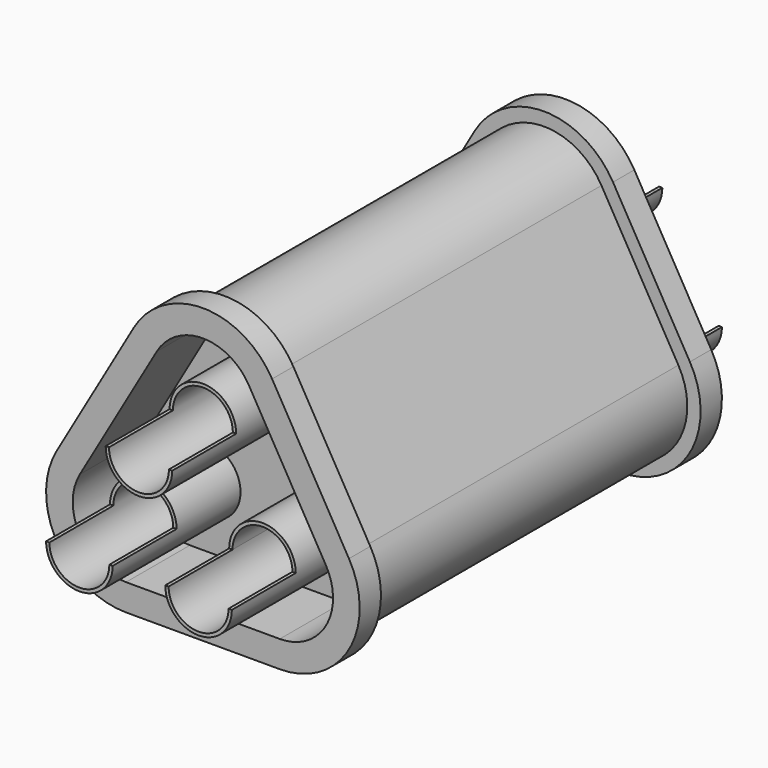
from build123d import *
from build123d import SkipClean  # not in build123d's __all__

# Parameters (mm, degrees)
F1_DEPTH  = 17
F2_DEPTH  = 1
F3_DEPTH  = 3
F4_DEPTH  = 17
F5_DEPTH  = 20
F6_DEPTH  = 14
F7_DEPTH  = 3
F8_DEPTH  = 3
F10_DEPTH = 1
F9_R      = 1.25
F11_DEPTH = 3


with BuildPart() as f1:
    # F0 (on Front) → F1 (new body)
    with BuildSketch(Plane.XZ):
        with BuildLine():
            Line((-2.1650635095, 3.4944827652), (-5.0518148554, -1.5055172348))
            ThreePointArc((-5.0518148554, -1.5055172348), (-5.0518148554, -4.0055172348), (-2.8867513459, -5.2555172348))
            Line((-2.8867513459, -5.2555172348), (2.8867513459, -5.2555172348))
            ThreePointArc((2.8867513459, -5.2555172348), (5.0518148554, -4.0055172348), (5.0518148554, -1.5055172348))
            Line((5.0518148554, -1.5055172348), (2.1650635095, 3.4944827652))
            ThreePointArc((2.1650635095, 3.4944827652), (0, 4.7444827652), (-2.1650635095, 3.4944827652))
        make_face()
        with BuildLine():
            ThreePointArc((-2.8867513459, -4.7555172348), (-4.6188021535, -3.7555172348), (-4.6188021535, -1.7555172348))
            Line((-4.6188021535, -1.7555172348), (-1.7320508076, 3.2444827652))
            ThreePointArc((-1.7320508076, 3.2444827652), (0, 4.2444827652), (1.7320508076, 3.2444827652))
            Line((1.7320508076, 3.2444827652), (4.6188021535, -1.7555172348))
            ThreePointArc((4.6188021535, -1.7555172348), (4.6188021535, -3.7555172348), (2.8867513459, -4.7555172348))
            Line((2.8867513459, -4.7555172348), (-2.8867513459, -4.7555172348))
        make_face(mode=Mode.SUBTRACT)
        with BuildLine():
            Line((-1.7320508076, 3.2444827652), (-4.6188021535, -1.7555172348))
            ThreePointArc((-4.6188021535, -1.7555172348), (-4.6188021535, -3.7555172348), (-2.8867513459, -4.7555172348))
            Line((-2.8867513459, -4.7555172348), (2.8867513459, -4.7555172348))
            ThreePointArc((2.8867513459, -4.7555172348), (4.6188021535, -3.7555172348), (4.6188021535, -1.7555172348))
            Line((4.6188021535, -1.7555172348), (1.7320508076, 3.2444827652))
            ThreePointArc((1.7320508076, 3.2444827652), (0, 4.2444827652), (-1.7320508076, 3.2444827652))
        make_face()
        with BuildLine():
            ThreePointArc((-3.4872322931, -2.3805172348), (-2.2372322931, -1.1305172348), (-0.9872322931, -2.3805172348))
            ThreePointArc((-0.9872322931, -2.3805172348), (-2.2372322931, -3.6305172348), (-3.4872322931, -2.3805172348))
        make_face(mode=Mode.SUBTRACT)
        with BuildLine():
            ThreePointArc((0.9872322931, -2.3805172348), (2.2372322931, -1.1305172348), (3.4872322931, -2.3805172348))
            ThreePointArc((3.4872322931, -2.3805172348), (2.2372322931, -3.6305172348), (0.9872322931, -2.3805172348))
        make_face(mode=Mode.SUBTRACT)
        with BuildLine():
            ThreePointArc((-1.25, 1.4944827652), (0, 2.7444827652), (1.25, 1.4944827652))
            ThreePointArc((1.25, 1.4944827652), (0, 0.2444827652), (-1.25, 1.4944827652))
        make_face(mode=Mode.SUBTRACT)
    extrude(amount=F1_DEPTH)

    # F0 (on Front) → F2 (join)
    with BuildSketch(Plane.XZ):
        with BuildLine():
            Line((-2.5980762114, 3.7444827652), (-5.4848275573, -1.2555172348))
            ThreePointArc((-5.4848275573, -1.2555172348), (-5.4848275573, -4.2555172348), (-2.8867513459, -5.7555172348))
            Line((-2.8867513459, -5.7555172348), (2.8867513459, -5.7555172348))
            ThreePointArc((2.8867513459, -5.7555172348), (5.4848275573, -4.2555172348), (5.4848275573, -1.2555172348))
            Line((5.4848275573, -1.2555172348), (2.5980762114, 3.7444827652))
            ThreePointArc((2.5980762114, 3.7444827652), (0, 5.2444827652), (-2.5980762114, 3.7444827652))
        make_face()
        with BuildLine():
            ThreePointArc((-2.8867513459, -5.2555172348), (-5.0518148554, -4.0055172348), (-5.0518148554, -1.5055172348))
            Line((-5.0518148554, -1.5055172348), (-2.1650635095, 3.4944827652))
            ThreePointArc((-2.1650635095, 3.4944827652), (0, 4.7444827652), (2.1650635095, 3.4944827652))
            Line((2.1650635095, 3.4944827652), (5.0518148554, -1.5055172348))
            ThreePointArc((5.0518148554, -1.5055172348), (5.0518148554, -4.0055172348), (2.8867513459, -5.2555172348))
            Line((2.8867513459, -5.2555172348), (-2.8867513459, -5.2555172348))
        make_face(mode=Mode.SUBTRACT)
    extrude(amount=F2_DEPTH)

    # F0 (on Front) → F3 (cut)
    with BuildSketch(Plane.XZ):
        with BuildLine():
            Line((-1.7320508076, 3.2444827652), (-4.6188021535, -1.7555172348))
            ThreePointArc((-4.6188021535, -1.7555172348), (-4.6188021535, -3.7555172348), (-2.8867513459, -4.7555172348))
            Line((-2.8867513459, -4.7555172348), (2.8867513459, -4.7555172348))
            ThreePointArc((2.8867513459, -4.7555172348), (4.6188021535, -3.7555172348), (4.6188021535, -1.7555172348))
            Line((4.6188021535, -1.7555172348), (1.7320508076, 3.2444827652))
            ThreePointArc((1.7320508076, 3.2444827652), (0, 4.2444827652), (-1.7320508076, 3.2444827652))
        make_face()
        with BuildLine():
            ThreePointArc((-3.4872322931, -2.3805172348), (-2.2372322931, -1.1305172348), (-0.9872322931, -2.3805172348))
            ThreePointArc((-0.9872322931, -2.3805172348), (-2.2372322931, -3.6305172348), (-3.4872322931, -2.3805172348))
        make_face(mode=Mode.SUBTRACT)
        with BuildLine():
            ThreePointArc((0.9872322931, -2.3805172348), (2.2372322931, -1.1305172348), (3.4872322931, -2.3805172348))
            ThreePointArc((3.4872322931, -2.3805172348), (2.2372322931, -3.6305172348), (0.9872322931, -2.3805172348))
        make_face(mode=Mode.SUBTRACT)
        with BuildLine():
            ThreePointArc((-1.25, 1.4944827652), (0, 2.7444827652), (1.25, 1.4944827652))
            ThreePointArc((1.25, 1.4944827652), (0, 0.2444827652), (-1.25, 1.4944827652))
        make_face(mode=Mode.SUBTRACT)
        with BuildLine():
            ThreePointArc((1.112232334, -2.3805172348), (2.2372322931, -3.5055171939), (3.3622322522, -2.3805172348))
            ThreePointArc((3.3622322522, -2.3805172348), (2.2372322931, -1.2555172756), (1.112232334, -2.3805172348))
        make_face()
        with BuildLine():
            ThreePointArc((-1.125, 1.4944827652), (0, 0.3694827652), (1.125, 1.4944827652))
            ThreePointArc((1.125, 1.4944827652), (0, 2.6194827652), (-1.125, 1.4944827652))
        make_face()
        with BuildLine():
            ThreePointArc((-3.3622322931, -2.3805172348), (-2.2372322931, -3.5055172348), (-1.1122322931, -2.3805172348))
            ThreePointArc((-1.1122322931, -2.3805172348), (-2.2372322931, -1.2555172348), (-3.3622322931, -2.3805172348))
        make_face()
    extrude(amount=F3_DEPTH, mode=Mode.SUBTRACT)

    # F9 (on face) → F10 (join)
    with BuildSketch(Plane.XZ.offset(17)):
        with BuildLine():
            Line((-2.5980762912, 3.7444828113), (-5.4848276371, -1.2555171887))
            ThreePointArc((-5.4848276371, -1.2555171887), (-5.4848276371, -4.2555172809), (-2.8867513459, -5.7555173269))
            Line((-2.8867513459, -5.7555173269), (2.8867513459, -5.7555173269))
            ThreePointArc((2.8867513459, -5.7555173269), (5.4848276371, -4.2555172809), (5.4848276371, -1.2555171887))
            Line((5.4848276371, -1.2555171887), (2.5980762912, 3.7444828113))
            ThreePointArc((2.5980762912, 3.7444828113), (0, 5.2444828574), (-2.5980762912, 3.7444828113))
        make_face()
        with BuildLine():
            Line((-5.0518148554, -1.5055172348), (-2.1650635095, 3.4944827652))
            ThreePointArc((-2.1650635095, 3.4944827652), (0, 4.7444827652), (2.1650635095, 3.4944827652))
            Line((2.1650635095, 3.4944827652), (5.0518148554, -1.5055172348))
            ThreePointArc((5.0518148554, -1.5055172348), (5.0518148554, -4.0055172348), (2.8867513459, -5.2555172348))
            Line((2.8867513459, -5.2555172348), (-2.8867513459, -5.2555172348))
            ThreePointArc((-2.8867513459, -5.2555172348), (-5.0518148554, -4.0055172348), (-5.0518148554, -1.5055172348))
        make_face(mode=Mode.SUBTRACT)
    extrude(amount=-F10_DEPTH)

    # F9 (on face) → F11 (cut)
    with BuildSketch(Plane.XZ.offset(17)):
        with BuildLine():
            Line((-1.7320508399, 3.2444827839), (-4.6188021858, -1.7555172161))
            ThreePointArc((-4.6188021858, -1.7555172161), (-4.6188021858, -3.7555172534), (-2.8867513459, -4.7555172721))
            Line((-2.8867513459, -4.7555172721), (2.8867513459, -4.7555172721))
            ThreePointArc((2.8867513459, -4.7555172721), (4.6188021858, -3.7555172534), (4.6188021858, -1.7555172161))
            Line((4.6188021858, -1.7555172161), (1.7320508399, 3.2444827839))
            ThreePointArc((1.7320508399, 3.2444827839), (0, 4.2444828025), (-1.7320508399, 3.2444827839))
        make_face()
        with Locations((-2.2372322931, -2.3805172348)):
            Circle(F9_R, mode=Mode.SUBTRACT)
        with Locations((2.2372322931, -2.3805172348)):
            Circle(F9_R, mode=Mode.SUBTRACT)
        with Locations((0, 1.4944827652)):
            Circle(F9_R, mode=Mode.SUBTRACT)
    extrude(amount=-F11_DEPTH, mode=Mode.SUBTRACT)


with BuildPart() as f4:
    # F0 (on Front) → F4 (new body)
    with BuildSketch(Plane.XZ):
        with BuildLine():
            Line((3.3622322522, -2.3805172348), (3.4872322931, -2.3805172348))
            ThreePointArc((3.4872322931, -2.3805172348), (2.2372322931, -1.1305172348), (0.9872322931, -2.3805172348))
            Line((0.9872322931, -2.3805172348), (1.112232334, -2.3805172348))
            ThreePointArc((1.112232334, -2.3805172348), (2.2372322931, -1.2555172756), (3.3622322522, -2.3805172348))
        make_face()
    extrude(amount=F4_DEPTH)

    # F0 (on Front) → F5 (join)
    with BuildSketch(Plane.XZ):
        with BuildLine():
            ThreePointArc((0.9872322931, -2.3805172348), (2.2372322931, -3.6305172348), (3.4872322931, -2.3805172348))
            Line((3.4872322931, -2.3805172348), (3.3622322522, -2.3805172348))
            ThreePointArc((3.3622322522, -2.3805172348), (2.2372322931, -3.5055171939), (1.112232334, -2.3805172348))
            Line((1.112232334, -2.3805172348), (0.9872322931, -2.3805172348))
        make_face()
    extrude(amount=F5_DEPTH)

    # F0 (on Front) → F6, piece 2 (join)
    with BuildSketch(Plane.XZ):
        with BuildLine():
            ThreePointArc((1.112232334, -2.3805172348), (2.2372322931, -3.5055171939), (3.3622322522, -2.3805172348))
            ThreePointArc((3.3622322522, -2.3805172348), (2.2372322931, -1.2555172756), (1.112232334, -2.3805172348))
        make_face()
    extrude(amount=F6_DEPTH)


with BuildPart() as f4b:
    # F0 (on Front) → F4, piece 2 (new body)
    with BuildSketch(Plane.XZ):
        with BuildLine():
            Line((1.125, 1.4944827652), (1.25, 1.4944827652))
            ThreePointArc((1.25, 1.4944827652), (0, 2.7444827652), (-1.25, 1.4944827652))
            Line((-1.25, 1.4944827652), (-1.125, 1.4944827652))
            ThreePointArc((-1.125, 1.4944827652), (0, 2.6194827652), (1.125, 1.4944827652))
        make_face()
    extrude(amount=F4_DEPTH)

    # F0 (on Front) → F5, piece 3 (join)
    with BuildSketch(Plane.XZ):
        with BuildLine():
            ThreePointArc((-1.25, 1.4944827652), (0, 0.2444827652), (1.25, 1.4944827652))
            Line((1.25, 1.4944827652), (1.125, 1.4944827652))
            ThreePointArc((1.125, 1.4944827652), (0, 0.3694827652), (-1.125, 1.4944827652))
            Line((-1.125, 1.4944827652), (-1.25, 1.4944827652))
        make_face()
    extrude(amount=F5_DEPTH)

    # F0 (on Front) → F6 (join)
    with BuildSketch(Plane.XZ):
        with BuildLine():
            ThreePointArc((-1.125, 1.4944827652), (0, 0.3694827652), (1.125, 1.4944827652))
            ThreePointArc((1.125, 1.4944827652), (0, 2.6194827652), (-1.125, 1.4944827652))
        make_face()
    extrude(amount=F6_DEPTH)


with BuildPart() as f4c:
    # F0 (on Front) → F4, piece 3 (new body)
    with BuildSketch(Plane.XZ):
        with BuildLine():
            Line((-1.1122322931, -2.3805172348), (-0.9872322931, -2.3805172348))
            ThreePointArc((-0.9872322931, -2.3805172348), (-2.2372322931, -1.1305172348), (-3.4872322931, -2.3805172348))
            Line((-3.4872322931, -2.3805172348), (-3.3622322931, -2.3805172348))
            ThreePointArc((-3.3622322931, -2.3805172348), (-2.2372322931, -1.2555172348), (-1.1122322931, -2.3805172348))
        make_face()
    extrude(amount=F4_DEPTH)

    # F0 (on Front) → F5, piece 2 (join)
    with BuildSketch(Plane.XZ):
        with BuildLine():
            ThreePointArc((-3.4872322931, -2.3805172348), (-2.2372322931, -3.6305172348), (-0.9872322931, -2.3805172348))
            Line((-0.9872322931, -2.3805172348), (-1.1122322931, -2.3805172348))
            ThreePointArc((-1.1122322931, -2.3805172348), (-2.2372322931, -3.5055172348), (-3.3622322931, -2.3805172348))
            Line((-3.3622322931, -2.3805172348), (-3.4872322931, -2.3805172348))
        make_face()
    extrude(amount=F5_DEPTH)

    # F0 (on Front) → F6, piece 3 (join)
    with BuildSketch(Plane.XZ):
        with BuildLine():
            ThreePointArc((-3.3622322931, -2.3805172348), (-2.2372322931, -3.5055172348), (-1.1122322931, -2.3805172348))
            ThreePointArc((-1.1122322931, -2.3805172348), (-2.2372322931, -1.2555172348), (-3.3622322931, -2.3805172348))
        make_face()
    extrude(amount=F6_DEPTH)


with BuildPart() as f7_tool:
    # F0 (on Front) → F7 (new body, through all)
    with BuildSketch(Plane.XZ):
        with BuildLine():
            ThreePointArc((-1.125, 1.4944827652), (0, 0.3694827652), (1.125, 1.4944827652))
            ThreePointArc((1.125, 1.4944827652), (0, 2.6194827652), (-1.125, 1.4944827652))
        make_face()
        with BuildLine():
            ThreePointArc((-3.3622322931, -2.3805172348), (-2.2372322931, -3.5055172348), (-1.1122322931, -2.3805172348))
            ThreePointArc((-1.1122322931, -2.3805172348), (-2.2372322931, -1.2555172348), (-3.3622322931, -2.3805172348))
        make_face()
        with BuildLine():
            ThreePointArc((1.112232334, -2.3805172348), (2.2372322931, -3.5055171939), (3.3622322522, -2.3805172348))
            ThreePointArc((3.3622322522, -2.3805172348), (2.2372322931, -1.2555172756), (1.112232334, -2.3805172348))
        make_face()
    extrude(amount=F7_DEPTH)


with BuildPart() as f4_1:
    add(f4.part, clean=False)

    # F7: cut by f7_tool
    add(f7_tool.part, mode=Mode.SUBTRACT)

    # F0 (on Front) → F8 (join)
    with BuildSketch(Plane.XZ):
        with BuildLine():
            ThreePointArc((0.9872322931, -2.3805172348), (2.2372322931, -3.6305172348), (3.4872322931, -2.3805172348))
            Line((3.4872322931, -2.3805172348), (3.3622322522, -2.3805172348))
            ThreePointArc((3.3622322522, -2.3805172348), (2.2372322931, -3.5055171939), (1.112232334, -2.3805172348))
            Line((1.112232334, -2.3805172348), (0.9872322931, -2.3805172348))
        make_face()
    with SkipClean():  # cleaning this boolean's faces spoils the solid; the shape is the same uncleaned
        extrude(amount=-F8_DEPTH)


with BuildPart() as f4b_1:
    add(f4b.part, clean=False)

    # F7: cut by f7_tool
    add(f7_tool.part, mode=Mode.SUBTRACT)

    # F0 (on Front) → F8, piece 3 (join)
    with BuildSketch(Plane.XZ):
        with BuildLine():
            ThreePointArc((-1.25, 1.4944827652), (0, 0.2444827652), (1.25, 1.4944827652))
            Line((1.25, 1.4944827652), (1.125, 1.4944827652))
            ThreePointArc((1.125, 1.4944827652), (0, 0.3694827652), (-1.125, 1.4944827652))
            Line((-1.125, 1.4944827652), (-1.25, 1.4944827652))
        make_face()
    extrude(amount=-F8_DEPTH)


with BuildPart() as f4c_1:
    add(f4c.part, clean=False)

    # F7: cut by f7_tool
    add(f7_tool.part, mode=Mode.SUBTRACT)

    # F0 (on Front) → F8, piece 2 (join)
    with BuildSketch(Plane.XZ):
        with BuildLine():
            ThreePointArc((-3.4872322931, -2.3805172348), (-2.2372322931, -3.6305172348), (-0.9872322931, -2.3805172348))
            Line((-0.9872322931, -2.3805172348), (-1.1122322931, -2.3805172348))
            ThreePointArc((-1.1122322931, -2.3805172348), (-2.2372322931, -3.5055172348), (-3.3622322931, -2.3805172348))
            Line((-3.3622322931, -2.3805172348), (-3.4872322931, -2.3805172348))
        make_face()
    with SkipClean():  # cleaning this boolean's faces spoils the solid; the shape is the same uncleaned
        extrude(amount=-F8_DEPTH)


solid = Compound([f1.part, f4_1.part, f4b_1.part, f4c_1.part])
